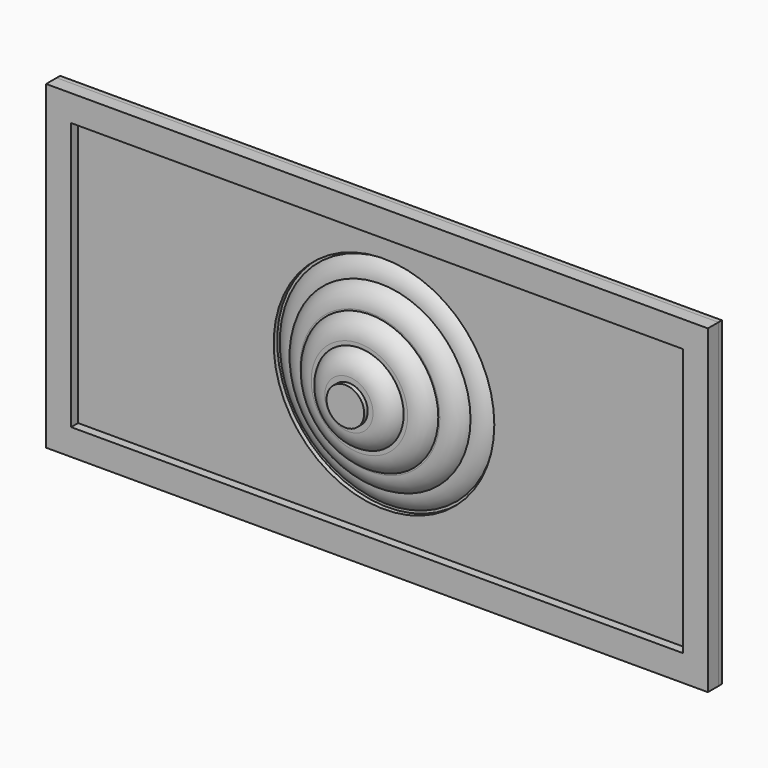
from build123d import *

# Parameters (mm, degrees)
F0_R      = 25.1181711361
F0_R_2    = 20.4995111856
F1_DEPTH  = 3
F0_R_3    = 15.560509686
F2_DEPTH  = 6
F0_R_4    = 10.0770984701
F3_DEPTH  = 9
F0_R_5    = 4.2848341216
F4_DEPTH  = 12
F0_R_6    = 1.2539122761
F5_DEPTH  = 13
F6_DEPTH  = 13
F0_W      = 150.6645679474
F0_H      = 72.9113966227
F0_W_2    = 139.2721533775
F0_H_2    = 60.949370265
F8_DEPTH  = 4
F9_DEPTH  = 2
F10_DEPTH = 1


# Not quite as in the source:
# - a fillet or chamfer that OpenCascade refuses, or shapes differently, is made with other operations: its cross-section is extruded or revolved along the edge and cut away or added


with BuildPart() as f1:
    # F0 (on Front) → F1 (new body)
    with BuildSketch(Plane.XZ):
        Circle(F0_R)
        Circle(F0_R_2, mode=Mode.SUBTRACT)
    extrude(amount=F1_DEPTH)

    # F0 (on Front) → F2 (join)
    with BuildSketch(Plane.XZ):
        Circle(F0_R_2)
        Circle(F0_R_3, mode=Mode.SUBTRACT)
    extrude(amount=F2_DEPTH)

    # F0 (on Front) → F3 (join)
    with BuildSketch(Plane.XZ):
        Circle(F0_R_3)
        Circle(F0_R_4, mode=Mode.SUBTRACT)
    extrude(amount=F3_DEPTH)

    # F0 (on Front) → F4 (join)
    with BuildSketch(Plane.XZ):
        Circle(F0_R_4)
        Circle(F0_R_5, mode=Mode.SUBTRACT)
    extrude(amount=F4_DEPTH)

    # F0 (on Front) → F5 (join)
    with BuildSketch(Plane.XZ):
        Circle(F0_R_5)
        Circle(F0_R_6, mode=Mode.SUBTRACT)
    extrude(amount=F5_DEPTH)

    # F0 (on Front) → F6 (join)
    with BuildSketch(Plane.XZ):
        Circle(F0_R_6)
    extrude(amount=F6_DEPTH)

    # F7: fillet of radius 5 on 4 edges, made by hand

    # F7_s1 → F7_t2 (revolve, cut)
    with BuildSketch(Plane.XY):
        with BuildLine():
            ThreePointArc((25.1181711361, 0), (23.2742082286, -2.1833001327), (20.5355954411, -3))
            Line((20.5355954411, -3), (25.1181711361, -3))
            Line((25.1181711361, -3), (25.1181711361, 0))
        make_face()
    revolve(axis=Axis((0, -3, 0), (0, -1, 0)), mode=Mode.SUBTRACT)

    # F7_s3 → F7_t4 (revolve, cut)
    with BuildSketch(Plane.XY):
        with BuildLine():
            ThreePointArc((20.4995111856, -3), (18.6555482782, -5.1833001327), (15.9169354907, -6))
            Line((15.9169354907, -6), (20.4995111856, -6))
            Line((20.4995111856, -6), (20.4995111856, -3))
        make_face()
    revolve(axis=Axis((0, -6, 0), (0, -1, 0)), mode=Mode.SUBTRACT)

    # F7_s5 → F7_t6 (revolve, cut)
    with BuildSketch(Plane.XY):
        with BuildLine():
            ThreePointArc((15.560509686, -6), (13.7165467785, -8.1833001327), (10.977933991, -9))
            Line((10.977933991, -9), (15.560509686, -9))
            Line((15.560509686, -9), (15.560509686, -6))
        make_face()
    revolve(axis=Axis((0, -9, 0), (0, -1, 0)), mode=Mode.SUBTRACT)

    # F7_s7 → F7_t8 (revolve, cut)
    with BuildSketch(Plane.XY):
        with BuildLine():
            ThreePointArc((10.0770984701, -9), (8.2331355627, -11.1833001327), (5.4945227752, -12))
            Line((5.4945227752, -12), (10.0770984701, -12))
            Line((10.0770984701, -12), (10.0770984701, -9))
        make_face()
    revolve(axis=Axis((0, -12, 0), (0, -1, 0)), mode=Mode.SUBTRACT)


with BuildPart() as f8:
    # F0 (on Front) → F8 (new body)
    with BuildSketch(Plane.XZ):
        Rectangle(F0_W, F0_H)
        Rectangle(F0_W_2, F0_H_2, mode=Mode.SUBTRACT)
    extrude(amount=F8_DEPTH)

    # F0 (on Front) → F9 (join)
    with BuildSketch(Plane.XZ):
        Rectangle(F0_W_2, F0_H_2)
        Circle(F0_R, mode=Mode.SUBTRACT)
    extrude(amount=F9_DEPTH)


with BuildPart() as f10:
    # F0 (on Front) → F10 (new body)
    with BuildSketch(Plane.XZ):
        Rectangle(F0_W, F0_H)
        Rectangle(F0_W_2, F0_H_2, mode=Mode.SUBTRACT)
        Rectangle(F0_W_2, F0_H_2)
        Circle(F0_R, mode=Mode.SUBTRACT)
        Circle(F0_R)
        Circle(F0_R_2, mode=Mode.SUBTRACT)
        Circle(F0_R_2)
        Circle(F0_R_3, mode=Mode.SUBTRACT)
        Circle(F0_R_3)
        Circle(F0_R_4, mode=Mode.SUBTRACT)
        Circle(F0_R_4)
        Circle(F0_R_5, mode=Mode.SUBTRACT)
        Circle(F0_R_5)
        Circle(F0_R_6, mode=Mode.SUBTRACT)
    extrude(amount=F10_DEPTH)


solid = Compound([f1.part, f8.part, f10.part])
